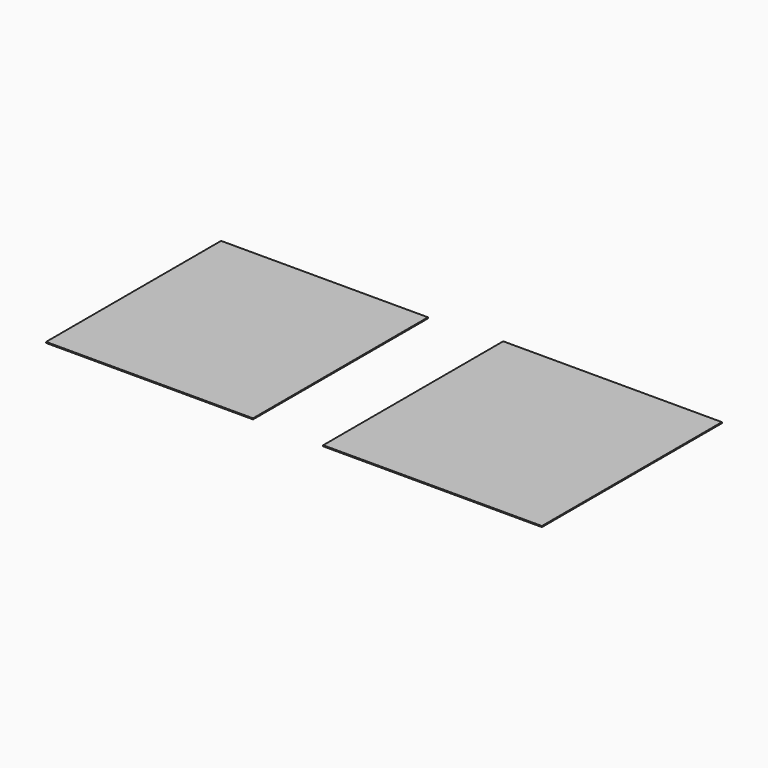
from build123d import *

# Parameters (mm, degrees)
F1_DEPTH = 2.032
F2_W     = 417.5125
F2_H     = 441.325
F3_DEPTH = 2.032


# Not quite as in the source:
# - a feature names something its author has since deleted; it is built from what else it names


with BuildPart() as f1:
    # F0 (on Top) → F1 (new body)
    with BuildSketch(Plane.XY):
        Polygon((217.4875, -227.0125), (220.6625, -227.0125), (220.6625, -144.4625), (220.6625, 227.0125), (-220.6625, 227.0125), (-220.6625, -144.4625), (-220.6625, -227.0125), (-217.4875, -227.0125), align=None)
    extrude(amount=F1_DEPTH)


with BuildPart() as f3:
    # F2 (on face) → F3 (new body)
    with BuildSketch(Plane.XY.offset(2.032)):
        with Locations((-570.6602515221, -6.7539259434)):
            Rectangle(F2_W, F2_H)
    extrude(amount=F3_DEPTH)


solid = Compound([f1.part, f3.part])
